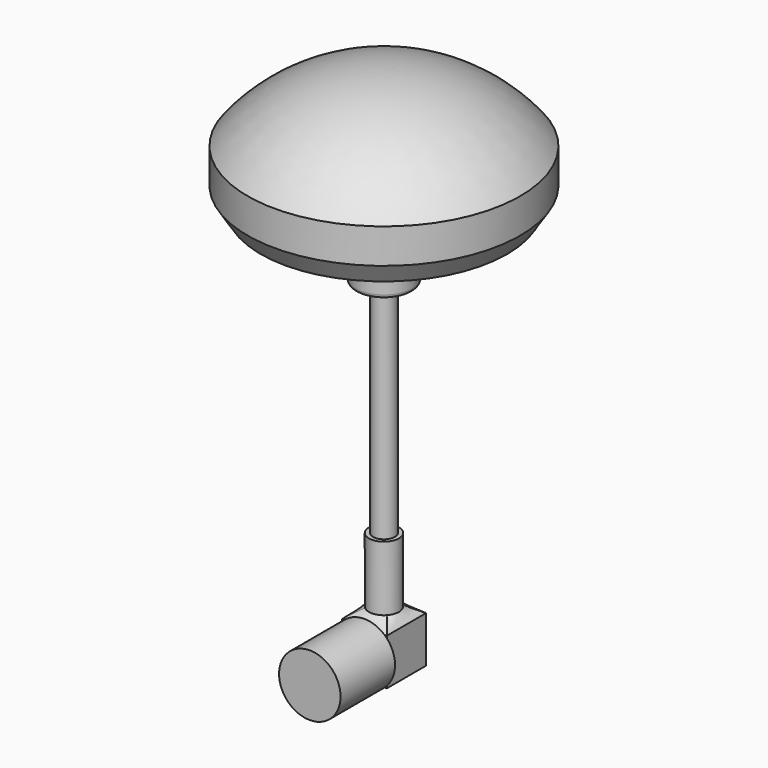
from build123d import *

# Parameters (mm, degrees)
F2_R      = 1.6
F3_DEPTH  = 32.4
F4_R      = 2.2
F5_DEPTH  = 9.5
F7_W      = 6.6
F7_H      = 7.2
F8_DEPTH  = 6.8
F8_FACE_W = 6.6
F8_FACE_H = 7.2
F10_R     = 4.51
F11_DEPTH = 10


# Not quite as in the source:
# - the arcs of a loft's sections are written as splines that run evenly, so that the points pair up as in the source's solid


with BuildPart() as f1:
    # F0 (on Right) → F1 (revolve)
    with BuildSketch(Plane.YZ):
        with BuildLine():
            Line((9.175, 0), (18.1, 0))
            Line((18.1, 0), (20, 3))
            Line((20, 3), (20, 8.1))
            ThreePointArc((20, 8.1), (11.1090613801, 15.1848660633), (0, 17.6))
            Line((0, 17.6), (0, -9.5))
            Line((0, -9.5), (3.675, -9.5))
            ThreePointArc((3.675, -9.5), (4.0285533906, -9.3535533906), (4.175, -9))
            Line((4.175, -9), (4.175, -5))
            ThreePointArc((4.175, -5), (5.6394660941, -1.4644660941), (9.175, 0))
        make_face()
    revolve(axis=Axis((0, 0, 4.05), (0, 0, 1)))

    # F2 (on face) → F3 (join)
    with BuildSketch(Plane(origin=(0, 0, -9.5), x_dir=(1, 0, 0), z_dir=(0, 0, -1))):
        Circle(F2_R)
    extrude(amount=F3_DEPTH)

    # F4 (on face) → F5 (join)
    with BuildSketch(Plane(origin=(0, 0, -41.9), x_dir=(1, 0, 0), z_dir=(0, 0, -1))):
        Circle(F4_R)
    extrude(amount=F5_DEPTH)



with BuildPart() as f8:
    # F7 (on offset) → F8 (new body)
    with BuildSketch(Plane(origin=(0, 0, -52.65), x_dir=(1, 0, 0), z_dir=(0, 0, -1))):
        Rectangle(F7_W, F7_H)
    extrude(amount=F8_DEPTH)


with BuildPart() as f1_1:
    add(f1.part)

    add(f8.part)  # F9 merges F8
    # F5_face (on face) → F9 section 0
    with BuildSketch(Plane(origin=(0, 0, -51.4), x_dir=(1, 0, 0), z_dir=(0, 0, -1))):
        with BuildLine():
            add(Edge.make_bspline(
                [(-1.4865941827, 1.6217391084), (-1.6988793356, 1.427144385), (-1.8723888959, 1.1904166981), (-2.1157043581, 0.6683765119), (-2.1854145258, 0.3832694131), (-2.210432571, -0.1921456263), (-2.165730605, -0.4822271657), (-1.9686424625, -1.0234153347), (-1.8163338319, -1.2743090299), (-1.6217391084, -1.4865941827)],
                knots=[0, 0, 0, 0, 0.25, 0.25, 0.5, 0.5, 0.75, 0.75, 1, 1, 1, 1], degree=3))
            add(Edge.make_bspline(
                [(-1.6217391084, -1.4865941827), (-1.427144385, -1.6988793356), (-1.1904166981, -1.8723888959), (-0.6683765119, -2.1157043581), (-0.3832694131, -2.1854145258), (0.1921456263, -2.210432571), (0.4822271657, -2.165730605), (1.0234153347, -1.9686424625), (1.2743090299, -1.8163338319), (1.4865941827, -1.6217391084)],
                knots=[0, 0, 0, 0, 0.25, 0.25, 0.5, 0.5, 0.75, 0.75, 1, 1, 1, 1], degree=3))
            add(Edge.make_bspline(
                [(1.4865941827, -1.6217391084), (1.6988793356, -1.427144385), (1.8723888959, -1.1904166981), (2.1157043581, -0.6683765119), (2.1854145258, -0.3832694131), (2.210432571, 0.1921456263), (2.165730605, 0.4822271657), (1.9686424625, 1.0234153347), (1.8163338319, 1.2743090299), (1.6217391084, 1.4865941827)],
                knots=[0, 0, 0, 0, 0.25, 0.25, 0.5, 0.5, 0.75, 0.75, 1, 1, 1, 1], degree=3))
            add(Edge.make_bspline(
                [(1.6217391084, 1.4865941827), (1.427144385, 1.6988793356), (1.1904166981, 1.8723888959), (0.6683765119, 2.1157043581), (0.3832694131, 2.1854145258), (-0.1921456263, 2.210432571), (-0.4822271657, 2.165730605), (-1.0234153347, 1.9686424625), (-1.2743090299, 1.8163338319), (-1.4865941827, 1.6217391084)],
                knots=[0, 0, 0, 0, 0.25, 0.25, 0.5, 0.5, 0.75, 0.75, 1, 1, 1, 1], degree=3))
        make_face()
    # F8_face (on face) → F9 section 1
    with BuildSketch(Plane.XY.offset(-52.65)):
        Rectangle(F8_FACE_W, F8_FACE_H)
    loft(ruled=True)

    # F10 (on face) → F11 (join)
    with BuildSketch(Plane.XZ.offset(3.6)):
        with Locations((0, -56.05)):
            Circle(F10_R)
    extrude(amount=F11_DEPTH)


solid = f1_1.part
